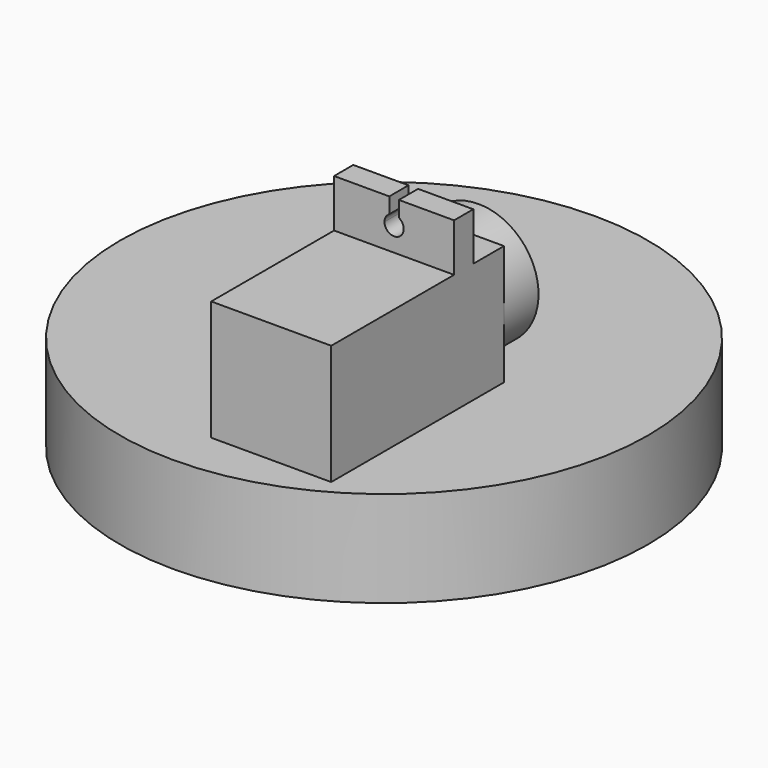
from build123d import *

# Parameters (mm, degrees)
F0_W      = 12.5
F0_H      = 22.5
F1_DEPTH  = 22.5
F2_W      = 12.5
F2_H      = 2.5
F3_DEPTH  = 5
F5_DEPTH  = 18.501
F7_DEPTH  = 4.5
F8_R      = 2.5
F8_R_2    = 1
F9_DEPTH  = 3
F11_R     = 27.5
F12_DEPTH = 10


# Not quite as in the source:
# - a pattern or mirror of a feature is missing from the dataset's text; its kind, count and spacing are read off the source's solid


with BuildPart() as f1:
    # F0 (on Top) → F1 (new body)
    with BuildSketch(Plane.XY):
        with Locations((6.25, -11.25)):
            Rectangle(F0_W, F0_H)
    extrude(amount=F1_DEPTH)

    # F2 (on face) → F3 (join)
    with BuildSketch(Plane.XY.offset(22.5)):
        with Locations((6.25, -5.25)):
            Rectangle(F2_W, F2_H)
    f3 = extrude(amount=F3_DEPTH)

    # F3_copies: F3 across plane
    add(f3.mirror(Plane(origin=(0, 0, 11.25), x_dir=(-1, 0, 0), z_dir=(0, 0, -1))))

    # F4 (on face) → F5 (cut, through all)
    with BuildSketch(Plane(origin=(0, -4, 0), x_dir=(-1, 0, 0), z_dir=(0, 1, 0))):
        with BuildLine():
            ThreePointArc((-6.75, 25.8660254038), (-6.75, 24.1339745962), (-5.25, 25))
            ThreePointArc((-5.25, 25), (-5.3839745962, 25.5), (-5.75, 25.8660254038))
            Line((-5.75, 25.8660254038), (-5.75, 25))
            Line((-5.75, 25), (-6.75, 25))
            Line((-6.75, 25), (-6.75, 25.8660254038))
        make_face()
        with BuildLine():
            Line((-5.75, 25), (-5.75, 25.8660254038))
            ThreePointArc((-5.75, 25.8660254038), (-6.25, 26), (-6.75, 25.8660254038))
            Line((-6.75, 25.8660254038), (-6.75, 25))
            Line((-6.75, 25), (-5.75, 25))
        make_face()
        with BuildLine():
            ThreePointArc((-6.75, 25.8660254038), (-6.25, 26), (-5.75, 25.8660254038))
            Line((-5.75, 25.8660254038), (-5.75, 27.5))
            Line((-5.75, 27.5), (-6.75, 27.5))
            Line((-6.75, 27.5), (-6.75, 25.8660254038))
        make_face()
    f5 = extrude(amount=-F5_DEPTH, mode=Mode.SUBTRACT)

    # F5_copies: F5 across plane
    add(f5.mirror(Plane(origin=(0, 0, 11.25), x_dir=(-1, 0, 0), z_dir=(0, 0, -1))), mode=Mode.SUBTRACT)

    # F6 (on face) → F7 (join)
    with BuildSketch(Plane(origin=(0, 0, 0), x_dir=(-1, 0, 0), z_dir=(0, 1, 0))):
        with BuildLine():
            ThreePointArc((-3.8005102572, 10.5), (-1.0359895046, 12.8037564576), (0, 16.25))
            ThreePointArc((0, 16.25), (-9.6962435424, 21.4640104954), (-8.6994897428, 10.5))
            ThreePointArc((-8.6994897428, 10.5), (-6.25, 12.5), (-3.8005102572, 10.5))
        make_face()
        with BuildLine():
            ThreePointArc((-3.8005102572, 10.5), (-6.25, 12.5), (-8.6994897428, 10.5))
            ThreePointArc((-8.6994897428, 10.5), (-6.25, 10), (-3.8005102572, 10.5))
        make_face()
        with BuildLine():
            ThreePointArc((-3.8005102572, 10.5), (-6.25, 10), (-8.6994897428, 10.5))
            ThreePointArc((-8.6994897428, 10.5), (-6.501272405, 7.5126596175), (-3.75, 10))
            ThreePointArc((-3.75, 10), (-3.7626596175, 10.251272405), (-3.8005102572, 10.5))
        make_face()
    extrude(amount=F7_DEPTH)

    # F8 (on face) → F9 (join)
    with BuildSketch(Plane(origin=(0, 4.5, 0), x_dir=(-1, 0, 0), z_dir=(0, 1, 0))):
        with Locations((-6.25, 16.25)):
            Circle(F8_R)
        with Locations((-6.25, 16.25)):
            Circle(F8_R_2, mode=Mode.SUBTRACT)
    extrude(amount=F9_DEPTH)


with BuildPart() as f12:
    # F11 (on Top) → F12 (new body)
    with BuildSketch(Plane.XY):
        Circle(F11_R)
    extrude(amount=F12_DEPTH)


solid = Compound([f1.part, f12.part])
